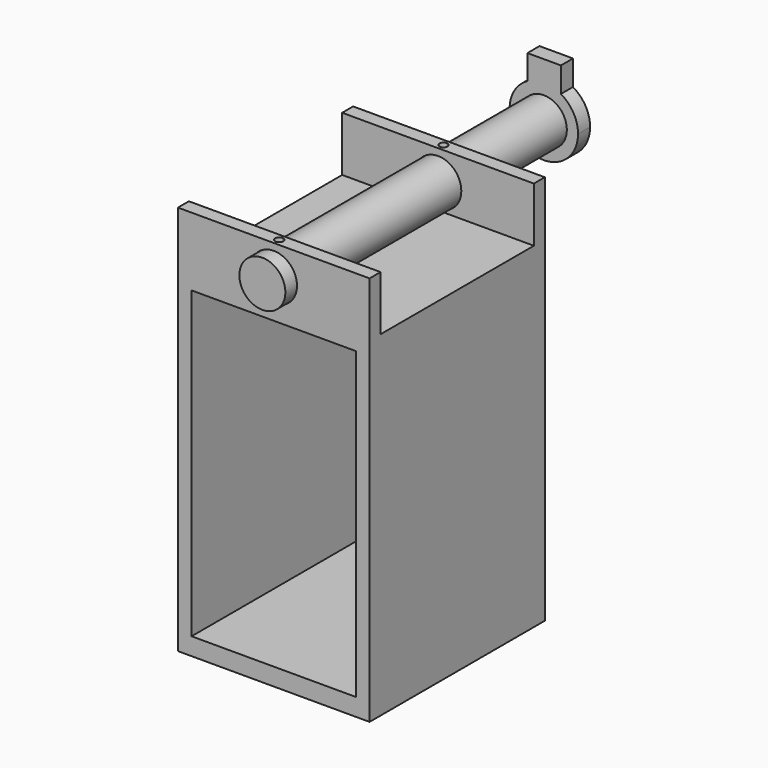
from build123d import *

# Parameters (mm, degrees)
F0_W      = 88.9
F0_H      = 101.6
F1_DEPTH  = 8.128
F2_W      = 6.35
F2_H      = 101.6
F3_DEPTH  = 141.224
F5_DEPTH  = 101.6
F6_W      = 88.9
F6_H      = 6.35
F7_DEPTH  = 25.4
F9_DEPTH  = 153.162
F10_R     = 10.668
F11_DEPTH = 108.204
F12_DEPTH = 61.976
F14_DEPTH = 7
F16_DEPTH = 7.62
F18_DEPTH = 7.62


with BuildPart() as f1:
    # F0 (on Top) → F1 (new body)
    with BuildSketch(Plane.XY):
        with Locations((7.6004267454, 38.7586035386)):
            Rectangle(F0_W, F0_H)
    extrude(amount=F1_DEPTH)

    # F2 (on face) → F3 (join)
    with BuildSketch(Plane.XY.offset(8.128)):
        with Locations((48.8754267454, 38.7586035386)):
            Rectangle(F2_W, F2_H)
        with Locations((-33.6745732546, 38.7586035386)):
            Rectangle(F2_W, F2_H)
    extrude(amount=F3_DEPTH)

    # F4 (on face) → F5 (join)
    with BuildSketch(Plane(origin=(0, 89.5586035386, 0), x_dir=(-1, 0, 0), z_dir=(0, 1, 0))):
        Polygon((-52.0504267454, 155.702), (-52.0504267454, 149.352), (-45.7004267454, 149.352), (30.4995732546, 149.352), (36.8495732546, 149.352), (36.8495732546, 155.702), align=None)
    extrude(amount=-F5_DEPTH)

    # F6 (on face) → F7 (join)
    with BuildSketch(Plane.XY.offset(155.702)):
        with Locations((7.6004267454, -8.8663964614)):
            Rectangle(F6_W, F6_H)
        with Locations((7.6004267454, 86.3836035386)):
            Rectangle(F6_W, F6_H)
    extrude(amount=F7_DEPTH)

    # F8 (on face) → F9 (cut)
    with BuildSketch(Plane(origin=(0, 89.5586035386, 0), x_dir=(-1, 0, 0), z_dir=(0, 1, 0))):
        with BuildLine():
            Line((-7.6004267454, 167.132), (3.1945732546, 167.132))
            ThreePointArc((3.1945732546, 167.132), (-7.6004267454, 177.927), (-18.3954267454, 167.132))
            Line((-18.3954267454, 167.132), (-7.6004267454, 167.132))
        make_face()
        with BuildLine():
            ThreePointArc((-18.3954267454, 167.132), (-7.6004267454, 156.337), (3.1945732546, 167.132))
            Line((3.1945732546, 167.132), (-7.6004267454, 167.132))
            Line((-7.6004267454, 167.132), (-18.3954267454, 167.132))
        make_face()
    extrude(amount=-F9_DEPTH, mode=Mode.SUBTRACT)

    # F15 (on face) → F16 (cut)
    with BuildSketch(Plane.XY.offset(181.102)):
        with BuildLine():
            ThreePointArc((9.5054267454, -8.8663964614), (8.9474651636, -7.5193580433), (7.6004267454, -6.9613964614))
            Line((7.6004267454, -6.9613964614), (7.6004267454, -10.7713964614))
            ThreePointArc((7.6004267454, -10.7713964614), (8.9474651636, -10.2134348796), (9.5054267454, -8.8663964614))
        make_face()
        with BuildLine():
            Line((7.6004267454, -10.7713964614), (7.6004267454, -6.9613964614))
            ThreePointArc((7.6004267454, -6.9613964614), (5.6954267454, -8.8663964614), (7.6004267454, -10.7713964614))
        make_face()
    extrude(amount=-F16_DEPTH, mode=Mode.SUBTRACT)

    # F17 (on face) → F18 (cut)
    with BuildSketch(Plane.XY.offset(181.102)):
        with BuildLine():
            ThreePointArc((9.5054267454, 86.3836035386), (8.9474651636, 87.7306419567), (7.6004267454, 88.2886035386))
            Line((7.6004267454, 88.2886035386), (7.6004267454, 84.4786035386))
            ThreePointArc((7.6004267454, 84.4786035386), (8.9474651636, 85.0365651204), (9.5054267454, 86.3836035386))
        make_face()
        with BuildLine():
            Line((7.6004267454, 84.4786035386), (7.6004267454, 88.2886035386))
            ThreePointArc((7.6004267454, 88.2886035386), (5.6954267454, 86.3836035386), (7.6004267454, 84.4786035386))
        make_face()
    extrude(amount=-F18_DEPTH, mode=Mode.SUBTRACT)


with BuildPart() as f11:
    # F10 (on face) → F11 (new body)
    with BuildSketch(Plane(origin=(0, 89.5586035386, 0), x_dir=(-1, 0, 0), z_dir=(0, 1, 0))):
        with Locations((-7.6004267454, 167.132)):
            Circle(F10_R)
    extrude(amount=-F11_DEPTH)

    # F12 (add): a face of the model
    f12_faces = [f11.faces().sort_by_distance(p)[0] for p in [
        (7.6004267454, 89.5586035386, 167.132),
    ]]
    extrude(f12_faces, amount=F12_DEPTH)


with BuildPart() as f14:
    # F13 (on face) → F14 (new body)
    with BuildSketch(Plane(origin=(0, 151.5346035386, 0), x_dir=(-1, 0, 0), z_dir=(0, 1, 0))):
        with BuildLine():
            Line((-18.2811267454, 167.132), (-23.4754267454, 167.132))
            ThreePointArc((-23.4754267454, 167.132), (-7.6004267454, 151.257), (8.2745732546, 167.132))
            Line((8.2745732546, 167.132), (3.0802732546, 167.132))
            ThreePointArc((3.0802732546, 167.132), (-7.6004267454, 156.4513), (-18.2811267454, 167.132))
        make_face()
        with BuildLine():
            ThreePointArc((-15.5379267454, 180.8801532851), (-21.3485800305, 175.0695), (-23.4754267454, 167.132))
            Line((-23.4754267454, 167.132), (-18.2811267454, 167.132))
            ThreePointArc((-18.2811267454, 167.132), (-17.5717709061, 170.9594858746), (-15.5379267454, 174.2785688439))
            Line((-15.5379267454, 174.2785688439), (-15.5379267454, 180.8801532851))
        make_face()
        with BuildLine():
            Line((0, 174.6360566214), (0, 181.069328951))
            ThreePointArc((0, 181.069328951), (-3.6786587829, 182.514956837), (-7.6004267454, 183.007))
            Line((-7.6004267454, 183.007), (-7.6004267454, 177.8127))
            ThreePointArc((-7.6004267454, 177.8127), (-3.4816420379, 176.9865910632), (0, 174.6360566214))
        make_face()
        with BuildLine():
            Line((3.0802732546, 167.132), (8.2745732546, 167.132))
            ThreePointArc((8.2745732546, 167.132), (6.0500750692, 175.2362843736), (0, 181.069328951))
            Line((0, 181.069328951), (0, 174.6360566214))
            ThreePointArc((0, 174.6360566214), (2.2802420181, 171.1878275697), (3.0802732546, 167.132))
        make_face()
        with BuildLine():
            ThreePointArc((-7.6004267454, 183.007), (-11.7091790864, 182.4660724923), (-15.5379267454, 180.8801532851))
            Line((-15.5379267454, 180.8801532851), (-15.5379267454, 174.2785688439))
            ThreePointArc((-15.5379267454, 174.2785688439), (-11.9447906021, 176.8892462903), (-7.6004267454, 177.8127))
            Line((-7.6004267454, 177.8127), (-7.6004267454, 183.007))
        make_face()
        with BuildLine():
            Line((-15.5379267454, 192.532), (-15.5379267454, 180.8801532851))
            ThreePointArc((-15.5379267454, 180.8801532851), (-11.7091790864, 182.4660724923), (-7.6004267454, 183.007))
            ThreePointArc((-7.6004267454, 183.007), (-3.6786587829, 182.514956837), (0, 181.069328951))
            Line((0, 181.069328951), (0, 192.532))
            Line((0, 192.532), (-15.5379267454, 192.532))
        make_face()
    extrude(amount=-F14_DEPTH)


solid = Compound([f1.part, f11.part, f14.part])
